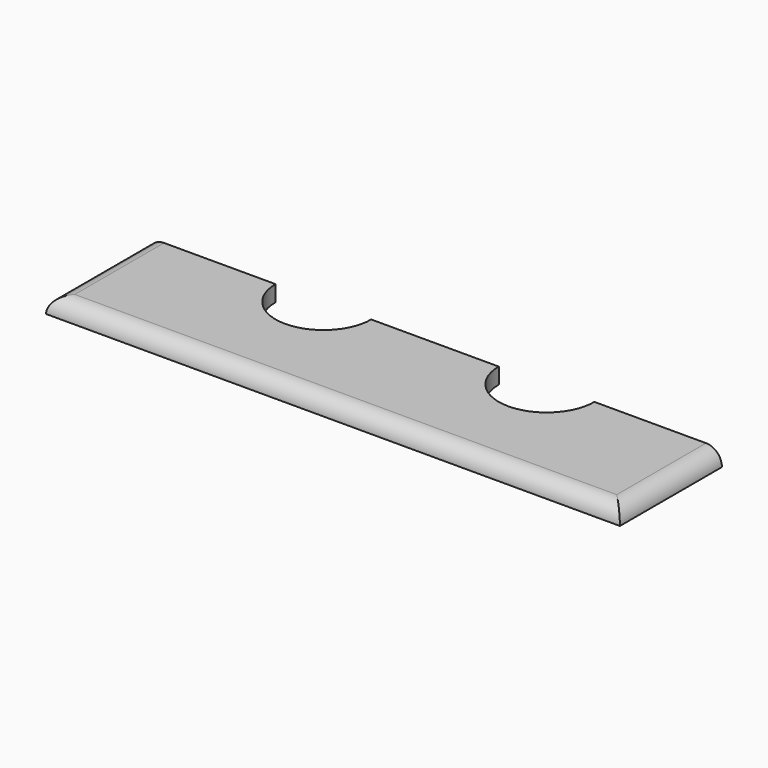
from build123d import *

# Parameters (mm, degrees)
F1_DEPTH = 5
F2_R     = 4.99999


# Not quite as in the source:
# - a fillet or chamfer is up to 0.001 mm smaller than in the source, because OpenCascade refuses the exact size


with BuildPart() as f1:
    # F0 (on Top) → F1 (new body)
    with BuildSketch(Plane.XY):
        with BuildLine():
            Line((20, 0), (0, 0))
            Line((0, 0), (-20, 0))
            ThreePointArc((-20, 0), (-35, -15), (-50, 0))
            Line((-50, 0), (-90, 0))
            Line((-90, 0), (-90, -40))
            Line((-90, -40), (0, -40))
            Line((0, -40), (90, -40))
            Line((90, -40), (90, 0))
            Line((90, 0), (50, 0))
            ThreePointArc((50, 0), (35, -15), (20, 0))
        make_face()
    extrude(amount=F1_DEPTH)

    # F2 (radius 5 in the source; OpenCascade refuses exactly that, so slightly less here)
    f2_edges = [f1.edges().sort_by_distance(p)[0] for p in [
        (0, -40, 5),
        (-90, -20, 5),
        (90, -20, 5),
    ]]
    fillet(f2_edges, radius=F2_R)


solid = f1.part
